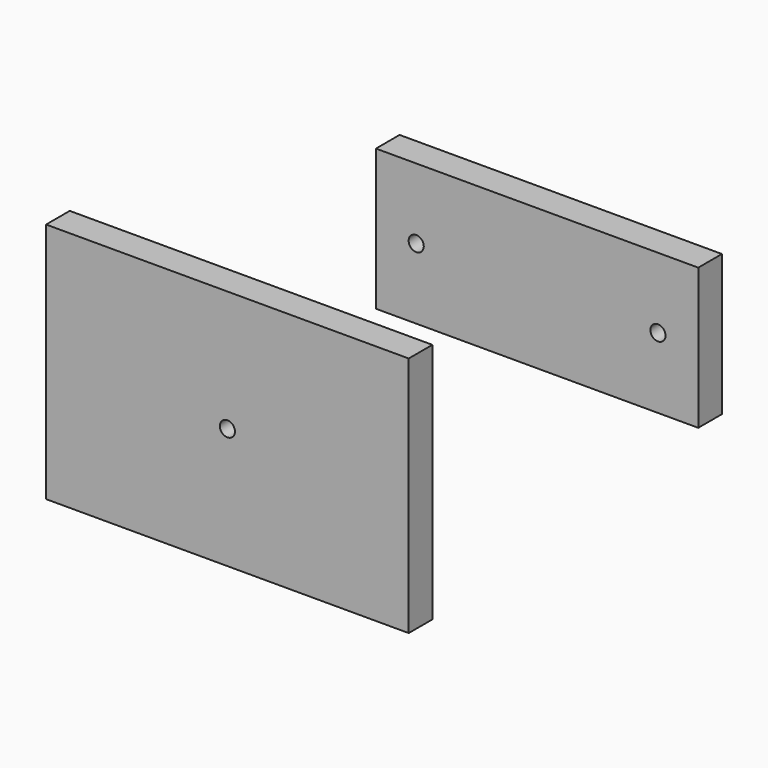
from build123d import *

# Parameters (mm, degrees)
F0_W     = 228.6
F0_H     = 18.6436
F4_DEPTH = 152.4
F1_R     = 4.7625
F2_DEPTH = 25.4
F3_DEPTH = 88.9
F0_W_2   = 50.8
F0_W_3   = 203.2
F5_R     = 4.7625
F6_DEPTH = 278.54900588


with BuildPart() as f4:
    # F0 (on Top) → F4 (new body)
    with BuildSketch(Plane.XY):
        with Locations((12.7, 22.0218)):
            Rectangle(F0_W, F0_H)
    extrude(amount=F4_DEPTH)

    # F1 (on face) → F2 (cut)
    with BuildSketch(Plane.XZ.offset(-12.7)):
        with Locations((12.7, 76.2)):
            Circle(F1_R)
    extrude(amount=-F2_DEPTH, mode=Mode.SUBTRACT)


with BuildPart() as f3:
    # F0 (on Top) → F3 (new body)
    with BuildSketch(Plane.XY):
        Polygon((-44.45, 62.6872), (-101.6, 62.6872), (-101.6, 44.0436), (-25.8064, 44.0436), align=None)
    extrude(amount=F3_DEPTH)


with BuildPart() as f3b:
    # F0 (on Top) → F3, piece 2 (new body)
    with BuildSketch(Plane.XY):
        with Locations((-76.2, 84.709)):
            Rectangle(F0_W_2, F0_H)
    extrude(amount=F3_DEPTH)


with BuildPart() as f3c:
    # F0 (on Top) → F3, piece 3 (new body)
    with BuildSketch(Plane.XY):
        with Locations((-76.2, 116.0526)):
            Rectangle(F0_W_2, F0_H)
    extrude(amount=F3_DEPTH)


with BuildPart() as f3d:
    # F0 (on Top) → F3, piece 4 (new body)
    with BuildSketch(Plane.XY):
        with Locations((0, 281.92620588)):
            Rectangle(F0_W_3, F0_H)
    extrude(amount=F3_DEPTH)

    # F5 (on face) → F6 (cut, through all)
    with BuildSketch(Plane(origin=(0, 291.24800588, 0), x_dir=(-1, 0, 0), z_dir=(0, 1, 0))):
        with Locations((76.2, 44.45)):
            Circle(F5_R)
        with Locations((-76.2, 44.45)):
            Circle(F5_R)
    extrude(amount=-F6_DEPTH, mode=Mode.SUBTRACT)


solid = Compound([f4.part, f3.part, f3b.part, f3c.part, f3d.part])
